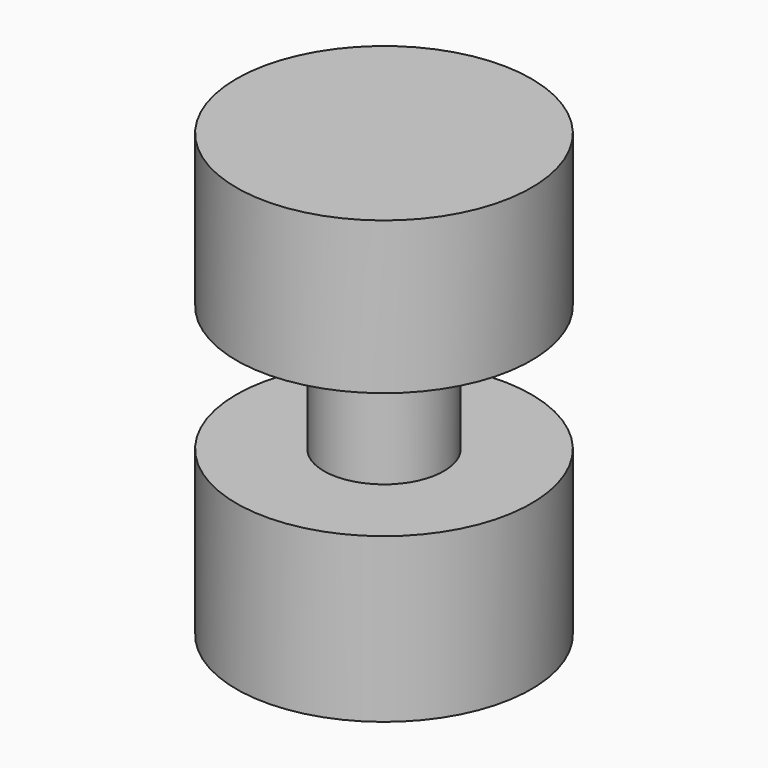
from build123d import *


with BuildPart() as f1:
    # F0 (on Front) → F1 (revolve)
    with BuildSketch(Plane.XZ):
        with BuildLine():
            ThreePointArc((-1.3, 1.772904835), (-1.2985563553, 3.2720701102), (0, 4.0212363124))
            Line((0, 4.0212363124), (0, 5))
            Line((0, 5), (-2.7067668361, 5))
            Line((-2.7067668361, 5), (-2.7067668361, 0))
            Line((-2.7067668361, 0), (-1.3, 0))
            Line((-1.3, 0), (-1.3, 1.772904835))
        make_face()
    revolve(axis=Axis((0, 0, 4.5106181562), (0, 0, -1)))

    # F4 (on Front) → F5 (revolve, cut)
    with BuildSketch(Plane.XZ):
        Polygon((0, 2.2098657209), (-1.4926502481, 2.2098657209), (-2.730937209, 2.2098657209), (-2.730937209, 0), (0, 0), align=None)
    revolve(axis=Axis((0, 0, 5), (0, 0, -1)), mode=Mode.SUBTRACT)


with BuildPart() as f3:
    # F2 (on Front) → F3 (revolve)
    with BuildSketch(Plane.XZ):
        with BuildLine():
            ThreePointArc((0, 3.8212363124), (-1.1381270623, 3.1494614233), (-1.1, 1.8284159893))
            Line((-1.1, 1.8284159893), (-1.1, -0.1))
            Line((-1.1, -0.1), (-2.7067668361, -0.1))
            Line((-2.7067668361, -0.1), (-2.7067668361, -3.1))
            Line((-2.7067668361, -3.1), (0, -3.1))
            Line((0, -3.1), (0, 0.2588959377))
            Line((0, 0.2588959377), (0, 3.8212363124))
        make_face()
    revolve(axis=Axis((0, 0, 0.3606181562), (0, 0, -1)))


solid = Compound([f1.part, f3.part])
